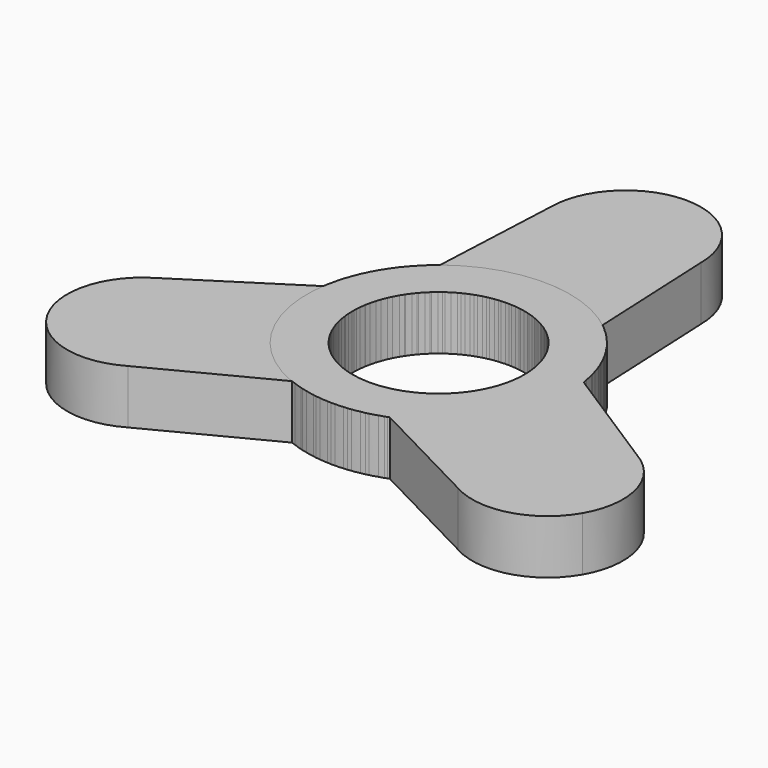
from build123d import *

# Parameters (mm, degrees)
F1_DEPTH        = 7
F1_COPIES_COUNT = 3


# Not quite as in the source:
# - a feature of the source that left no trace in its solid (it failed there, or was rolled back) is left out
# - a pattern or mirror of a feature is missing from the dataset's text; its kind, count and spacing are read off the source's solid
# - the program builds the solid bodies; features that only make, move or delete a surface that nothing else refers to are left out


with BuildPart() as f1:
    # F0 (on Top) → F1 (new body)
    with BuildSketch(Plane.XY):
        with BuildLine():
            ThreePointArc((11.1131159341, 0.5140809622), (11.1220285867, 0.2571091533), (11.125, 0))
            ThreePointArc((11.125, 0), (-0.2571092012, -11.1220285856), (-11.1131159296, 0.514081058))
            Line((-11.1131159296, 0.514081058), (-10.5178425687, 13.3823612856))
            ThreePointArc((-10.5178425687, 13.3823612856), (-7.4393875591, -15.3090861459), (17.0209460923, 0))
            ThreePointArc((17.0209460923, 0), (15.3090861459, 7.4393875591), (10.5178425687, 13.3823612856))
            Line((10.5178425687, 13.3823612856), (11.1131159341, 0.5140809622))
        make_face()
        with BuildLine():
            Line((-10.5178425687, 13.3823612856), (-11.1131159296, 0.514081058))
            ThreePointArc((-11.1131159296, 0.514081058), (-7.6826581738, 8.0462654931), (0, 11.125))
            Line((0, 11.125), (0, 17.0209460923))
            ThreePointArc((0, 17.0209460923), (-5.5647172366, 16.0856000184), (-10.5178425687, 13.3823612856))
        make_face()
        with BuildLine():
            ThreePointArc((0, 11.125), (7.6826582084, 8.04626546), (11.1131159341, 0.5140809622))
            Line((11.1131159341, 0.5140809622), (10.5178425687, 13.3823612856))
            ThreePointArc((10.5178425687, 13.3823612856), (5.5647172366, 16.0856000184), (0, 17.0209460923))
            Line((0, 17.0209460923), (0, 11.125))
        make_face()
        with BuildLine():
            ThreePointArc((0, 17.0209460923), (5.5647172366, 16.0856000184), (10.5178425687, 13.3823612856))
            Line((10.5178425687, 13.3823612856), (9.7369597852, 30.2630402148))
            ThreePointArc((9.7369597852, 30.2630402148), (6.8850702923, 23.3779699225), (0, 20.5260804296))
            Line((0, 20.5260804296), (0, 17.0209460923))
        make_face()
        with BuildLine():
            ThreePointArc((0, 20.5260804296), (6.8850702923, 23.3779699225), (9.7369597852, 30.2630402148))
            Line((9.7369597852, 30.2630402148), (0, 30.2630402148))
            Line((0, 30.2630402148), (0, 20.5260804296))
        make_face()
        with BuildLine():
            Line((-9.7369597852, 30.2630402148), (-10.5178425687, 13.3823612856))
            ThreePointArc((-10.5178425687, 13.3823612856), (-5.5647172366, 16.0856000184), (0, 17.0209460923))
            Line((0, 17.0209460923), (0, 20.5260804296))
            ThreePointArc((0, 20.5260804296), (-6.8850702923, 23.3779699225), (-9.7369597852, 30.2630402148))
        make_face()
        with BuildLine():
            ThreePointArc((0, 40), (-6.8850702923, 37.148110507), (-9.7369597852, 30.2630402148))
            Line((-9.7369597852, 30.2630402148), (0, 30.2630402148))
            Line((0, 30.2630402148), (0, 40))
        make_face()
        with BuildLine():
            Line((0, 30.2630402148), (9.7369597852, 30.2630402148))
            ThreePointArc((9.7369597852, 30.2630402148), (6.8850702923, 37.148110507), (0, 40))
            Line((0, 40), (0, 30.2630402148))
        make_face()
        with BuildLine():
            Line((0, 30.2630402148), (-9.7369597852, 30.2630402148))
            ThreePointArc((-9.7369597852, 30.2630402148), (-6.8850702923, 23.3779699225), (0, 20.5260804296))
            Line((0, 20.5260804296), (0, 30.2630402148))
        make_face()
    extrude(amount=F1_DEPTH)


with BuildPart() as f1_copies_1:
    # F1_copies: instance of F1
    add(f1.part.rotate(Axis((0, 0, 0), (0, 0, 1)), 1 * 360 / F1_COPIES_COUNT))


with BuildPart() as f1_copies_2:
    # F1_copies: instance of F1
    add(f1.part.rotate(Axis((0, 0, 0), (0, 0, 1)), 2 * 360 / F1_COPIES_COUNT))


solid = Compound([f1.part, f1_copies_1.part, f1_copies_2.part])
